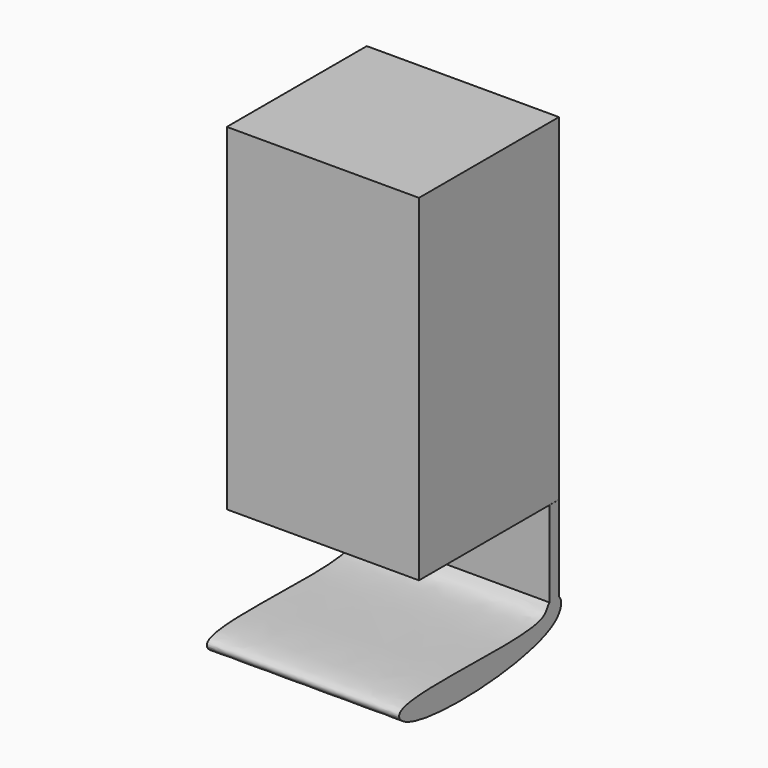
from build123d import *

# Parameters (mm, degrees)
F0_W     = 73.4944455326
F0_H     = 128.8070529699
F1_DEPTH = 66.91422
F3_DEPTH = 73.52671
F4_R     = 13.0714114786
F5_DEPTH = 25.4


with BuildPart() as f1:
    # F0 (on Front) → F1 (new body)
    with BuildSketch(Plane.XZ):
        with Locations((0.3371294588, -11.3651156425)):
            Rectangle(F0_W, F0_H)
    extrude(amount=F1_DEPTH)

    # F4 (on face) → F5 (cut)
    with BuildSketch(Plane(origin=(0, 0, -75.7686421275), x_dir=(1, 0, 0), z_dir=(0, 0, -1))):
        with Locations((0, 28.8865305483)):
            Circle(F4_R)
    extrude(amount=-F5_DEPTH, mode=Mode.SUBTRACT)


with BuildPart() as f3:
    # F2 (on face) → F3 (new body)
    with BuildSketch(Plane(origin=(-36.4100933075, 0, 0), x_dir=(0, -1, 0), z_dir=(-1, 0, 0))):
        with BuildLine():
            Line((4.5693493448, -75.7686421275), (0, -75.7686421275))
            Line((0, -75.7686421275), (0, -108.5322573781))
            add(Edge.make_bspline(
                [(4.5693493448, -108.5322573781), (3.4544405111, -107.6442845671), (1.2443930447, -107.4803571585), (0, -108.5322573781)],
                knots=[0.9192317518, 0.9192317518, 0.9192317518, 0.9192317518, 1, 1, 1, 1], degree=3))
            Line((4.5693493448, -108.5322573781), (4.5693493448, -75.7686421275))
        make_face()
        with BuildLine():
            add(Edge.make_bspline(
                [(4.5693493448, -108.5322573781), (3.4544405111, -107.6442845671), (1.2443930447, -107.4803571585), (0, -108.5322573781)],
                knots=[0.9192317518, 0.9192317518, 0.9192317518, 0.9192317518, 1, 1, 1, 1], degree=3))
            add(Edge.make_bspline(
                [(0, -108.5322573781), (-1.6612931093, -109.9365681736), (-1.4264246437, -123.9678277985), (71.1222384867, -127.3478206349), (82.6559450921, -110.1035008934), (5.1463672701, -118.0822262935), (5.8483480225, -109.5509200855), (4.5693493448, -108.5322573781)],
                knots=[0, 0, 0, 0, 0.1078274543, 0.4236470104, 0.5182856205, 0.8265762096, 0.9192317518, 0.9192317518, 0.9192317518, 0.9192317518], degree=3))
        make_face()
    extrude(amount=-F3_DEPTH)


solid = Compound([f1.part, f3.part])
